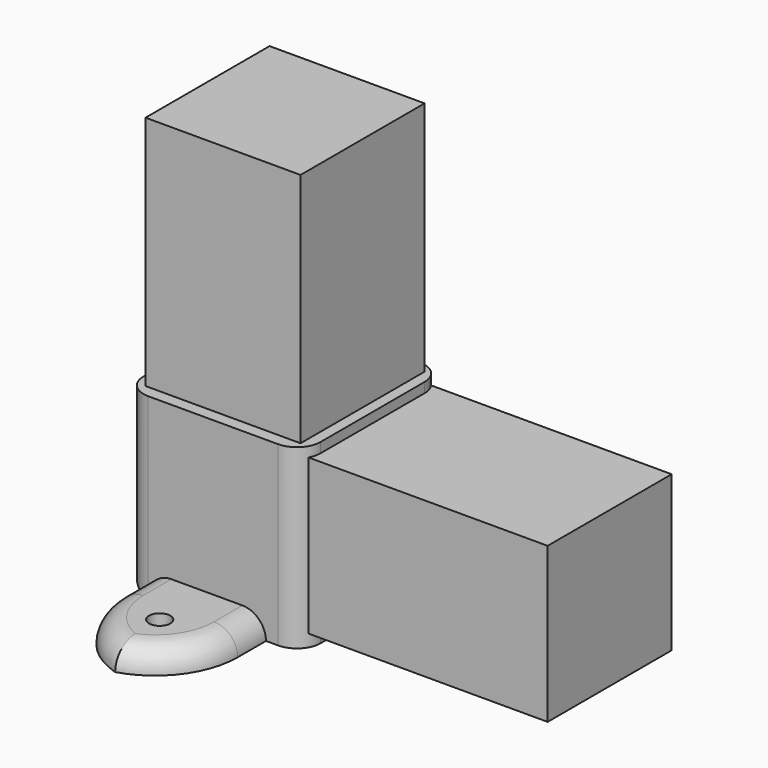
from build123d import *

# Parameters (mm, degrees)
F0_W           = 38.1
F0_H           = 38.1
F1_DEPTH       = 38.1
F2_W           = 33.3375
F2_H           = 33.3375
F3_DEPTH       = 50.8
F4_W           = 33.3375
F4_H           = 33.3375
F5_DEPTH       = 50.8
F6_W           = 25.4
F6_H           = 25.4
F7_DEPTH       = 5.08
F8_R           = 2.286
F9_DEPTH       = 83.82
F10_T1_DEPTH   = 93.9954855022
F10_2_T1_DEPTH = 93.9954855022
F11_T1_DEPTH   = 63.5
F11_T3_DEPTH   = 63.5
F11_T8_DEPTH   = 63.5
F11_T14_DEPTH  = 63.5
F11_T20_DEPTH  = 63.5
F11_T27_DEPTH  = 63.5
F11_T33_DEPTH  = 63.5
F11_T39_DEPTH  = 63.5
F11_T45_DEPTH  = 63.5
F11_T51_DEPTH  = 63.5
F11_T58_DEPTH  = 63.5
F11_T64_DEPTH  = 63.5
F11_2_T1_DEPTH = 20.3169028996
F11_2_T4_ANGLE = 114.3203710668
F11_2_T6_ANGLE = 114.3203710677
F11_3_T1_DEPTH = 20.3169028996
F11_3_T4_ANGLE = 114.3203710668
F11_3_T6_ANGLE = 114.3203710677


# Not quite as in the source:
# - a fillet or chamfer that OpenCascade refuses, or shapes differently, is made with other operations: its cross-section is extruded or revolved along the edge and cut away or added


with BuildPart() as f1:
    # F0 (on Front) → F1 (new body)
    with BuildSketch(Plane.XZ):
        with Locations((19.3985427063, -10.1599991322)):
            Rectangle(F0_W, F0_H)
    extrude(amount=F1_DEPTH)

    # F2 (on face) → F3 (join)
    with BuildSketch(Plane.YZ.offset(38.4485427063)):
        with Locations((-18.8190903282, -9.9104456074)):
            Rectangle(F2_W, F2_H)
    extrude(amount=F3_DEPTH)

    # F11: fillet of radius 5.08 on 5 edges, made by hand

    # F11_s2 → F11_t1 (cut)
    with BuildSketch(Plane.XY.offset(-41.9099991322)):
        with BuildLine():
            ThreePointArc((0.3485427063, -5.08), (1.8364402579, -1.4878975516), (5.4285427063, 0))
            Line((5.4285427063, 0), (0.3485427063, 0))
            Line((0.3485427063, 0), (0.3485427063, -5.08))
        make_face()
        with BuildLine():
            ThreePointArc((0.3485427063, -33.02), (1.8364402579, -36.6121024484), (5.4285427063, -38.1))
            Line((5.4285427063, -38.1), (0.3485427063, -38.1))
            Line((0.3485427063, -38.1), (0.3485427063, -33.02))
        make_face()
    extrude(amount=F11_T1_DEPTH, mode=Mode.SUBTRACT)

    # F11_s4 → F11_t3 (cut)
    with BuildSketch(Plane.XZ.offset(-12.7)):
        with BuildLine():
            ThreePointArc((0.3485427063, -24.1299991322), (1.8364402579, -27.7221015806), (5.4285427063, -29.2099991322))
            Line((5.4285427063, -29.2099991322), (0.3485427063, -29.2099991322))
            Line((0.3485427063, -29.2099991322), (0.3485427063, -24.1299991322))
        make_face()
    extrude(amount=F11_T3_DEPTH, mode=Mode.SUBTRACT)


with BuildPart() as f5:
    # F4 (on face) → F5 (new body)
    with BuildSketch(Plane.XY.offset(8.8900008678)):
        with Locations((19.4469346859, -18.8190890476)):
            Rectangle(F4_W, F4_H)
    extrude(amount=F5_DEPTH)


with BuildPart() as f7:
    # F6 (on face) → F7 (new body)
    with BuildSketch(Plane(origin=(0, 0, -29.2099991322), x_dir=(1, 0, 0), z_dir=(0, 0, -1))):
        with Locations((18.0697256371, -12.7)):
            Rectangle(F6_W, F6_H)
    extrude(amount=-F7_DEPTH)


with BuildPart() as f7b:
    # F6 (on face) → F7, piece 2 (new body)
    with BuildSketch(Plane(origin=(0, 0, -29.2099991322), x_dir=(1, 0, 0), z_dir=(0, 0, -1))):
        with Locations((18.0697256371, 50.8)):
            Rectangle(F6_W, F6_H)
    extrude(amount=-F7_DEPTH)


with BuildPart() as f9_tool:
    # F8 (on face) → F9 (new body)
    with BuildSketch(Plane.XY.offset(-24.1299991322)):
        with Locations((18.0697256371, -50.8)):
            Circle(F8_R)
        with Locations((18.0697256371, 12.7)):
            Circle(F8_R)
    extrude(amount=-F9_DEPTH)


with BuildPart() as f7_1:
    add(f7.part)

    # F9: cut by f9_tool
    add(f9_tool.part, mode=Mode.SUBTRACT)

    # F10: fillet of radius 17.7830971004 on 2 edges, made by hand

    # F10_s2 → F10_t1 (cut)
    with BuildSketch(Plane.XY.offset(-73.6677418833)):
        with BuildLine():
            ThreePointArc((5.3697256371, 7.6169028996), (10.5782741874, 20.1914514498), (23.1528227376, 25.4))
            Line((23.1528227376, 25.4), (5.3697256371, 25.4))
            Line((5.3697256371, 25.4), (5.3697256371, 7.6169028996))
        make_face()
        with BuildLine():
            ThreePointArc((30.7697256371, 7.6169028996), (25.5611770869, 20.1914514498), (12.9866285367, 25.4))
            Line((12.9866285367, 25.4), (30.7697256371, 25.4))
            Line((30.7697256371, 25.4), (30.7697256371, 7.6169028996))
        make_face()
    extrude(amount=F10_T1_DEPTH, mode=Mode.SUBTRACT)

    # F11#2: fillet of radius 5.08 on 2 edges, made by hand

    # F11_2_s2 → F11_2_t1 (cut)
    with BuildSketch(Plane.XZ.offset(-7.6169028996)):
        with BuildLine():
            ThreePointArc((30.7697256371, -29.2099991322), (29.2818280856, -25.6178966837), (25.6897256371, -24.1299991322))
            Line((25.6897256371, -24.1299991322), (30.7697256371, -24.1299991322))
            Line((30.7697256371, -24.1299991322), (30.7697256371, -29.2099991322))
        make_face()
        with BuildLine():
            ThreePointArc((5.3697256371, -29.2099991322), (6.8576231887, -25.6178966837), (10.4497256371, -24.1299991322))
            Line((10.4497256371, -24.1299991322), (5.3697256371, -24.1299991322))
            Line((5.3697256371, -24.1299991322), (5.3697256371, -29.2099991322))
        make_face()
    extrude(amount=F11_2_T1_DEPTH, mode=Mode.SUBTRACT)

    # F11_2_s3 → F11_2_t4 (revolve, cut)
    with BuildSketch(Plane.XZ.offset(-7.6169028995)):
        with BuildLine():
            ThreePointArc((10.4497256371, -24.1299991322), (6.8576231887, -25.6178966837), (5.3697256371, -29.2099991322))
            Line((5.3697256371, -29.2099991322), (5.3697256371, -24.1299991322))
            Line((5.3697256371, -24.1299991322), (10.4497256371, -24.1299991322))
        make_face()
    revolve(axis=Axis((23.1528227376, 7.6169028995, -24.1299991322), (0, 0, -1)), revolution_arc=F11_2_T4_ANGLE, mode=Mode.SUBTRACT)

    # F11_2_s5 → F11_2_t6 (revolve, cut)
    with BuildSketch(Plane(origin=(13.6425072573, 6.165668504, 0), x_dir=(0, 0, 1), z_dir=(-0.9112569083, -0.4118383749, 0))):
        with BuildLine():
            ThreePointArc((-24.1299991322, 14.2956604954), (-25.6178966837, 17.8877629438), (-29.2099991322, 19.3756604954))
            Line((-29.2099991322, 19.3756604954), (-24.1299991322, 19.3756604954))
            Line((-24.1299991322, 19.3756604954), (-24.1299991322, 14.2956604954))
        make_face()
    revolve(axis=Axis((12.9866285367, 7.6169028996, -24.1299991322), (0, 0, -1)), revolution_arc=F11_2_T6_ANGLE, mode=Mode.SUBTRACT)


with BuildPart() as f7b_1:
    add(f7b.part)

    # F9: cut by f9_tool
    add(f9_tool.part, mode=Mode.SUBTRACT)

    # F10#2: fillet of radius 17.7830971004 on 2 edges, made by hand

    # F10_2_s2 → F10_2_t1 (cut)
    with BuildSketch(Plane.XY.offset(-73.6677418833)):
        with BuildLine():
            ThreePointArc((23.1528227376, -63.5), (10.5782741874, -58.2914514498), (5.3697256371, -45.7169028996))
            Line((5.3697256371, -45.7169028996), (5.3697256371, -63.5))
            Line((5.3697256371, -63.5), (23.1528227376, -63.5))
        make_face()
        with BuildLine():
            ThreePointArc((12.9866285367, -63.5), (25.5611770869, -58.2914514498), (30.7697256371, -45.7169028996))
            Line((30.7697256371, -45.7169028996), (30.7697256371, -63.5))
            Line((30.7697256371, -63.5), (12.9866285367, -63.5))
        make_face()
    extrude(amount=F10_2_T1_DEPTH, mode=Mode.SUBTRACT)

    # F11#3: fillet of radius 5.08 on 2 edges, made by hand

    # F11_3_s2 → F11_3_t1 (cut)
    with BuildSketch(Plane.XZ.offset(25.4)):
        with BuildLine():
            ThreePointArc((30.7697256371, -29.2099991322), (29.2818280856, -25.6178966837), (25.6897256371, -24.1299991322))
            Line((25.6897256371, -24.1299991322), (30.7697256371, -24.1299991322))
            Line((30.7697256371, -24.1299991322), (30.7697256371, -29.2099991322))
        make_face()
        with BuildLine():
            ThreePointArc((10.4497256371, -24.1299991322), (6.8576231887, -25.6178966837), (5.3697256371, -29.2099991322))
            Line((5.3697256371, -29.2099991322), (5.3697256371, -24.1299991322))
            Line((5.3697256371, -24.1299991322), (10.4497256371, -24.1299991322))
        make_face()
    extrude(amount=F11_3_T1_DEPTH, mode=Mode.SUBTRACT)

    # F11_3_s3 → F11_3_t4 (revolve, cut)
    with BuildSketch(Plane(origin=(2.0687305768, 0.9349532839, 0), x_dir=(0, 0, 1), z_dir=(0.9112569083, 0.4118383749, 0))):
        with BuildLine():
            ThreePointArc((-24.1299991322, 63.8981615853), (-25.6178966837, 67.4902640337), (-29.2099991322, 68.9781615853))
            Line((-29.2099991322, 68.9781615853), (-24.1299991322, 68.9781615853))
            Line((-24.1299991322, 68.9781615853), (-24.1299991322, 63.8981615853))
        make_face()
    revolve(axis=Axis((23.1528227376, -45.7169028995, -24.1299991322), (0, 0, -1)), revolution_arc=F11_3_T4_ANGLE, mode=Mode.SUBTRACT)

    # F11_3_s5 → F11_3_t6 (revolve, cut)
    with BuildSketch(Plane.XZ.offset(45.7169028996)):
        with BuildLine():
            ThreePointArc((30.7697256371, -29.2099991322), (29.2818280855, -25.6178966837), (25.6897256371, -24.1299991322))
            Line((25.6897256371, -24.1299991322), (30.7697256371, -24.1299991322))
            Line((30.7697256371, -24.1299991322), (30.7697256371, -29.2099991322))
        make_face()
    revolve(axis=Axis((12.9866285367, -45.7169028996, -24.1299991322), (0, 0, -1)), revolution_arc=F11_3_T6_ANGLE, mode=Mode.SUBTRACT)


with BuildPart() as f11_tool6:
    # F11_s7 → F11_t8 (new body)
    with BuildSketch(Plane.XY.offset(-41.9099991322)):
        with BuildLine():
            ThreePointArc((38.4485427063, -5.08), (36.9606451548, -1.4878975516), (33.3685427063, 0))
            Line((33.3685427063, 0), (38.4485427063, 0))
            Line((38.4485427063, 0), (38.4485427063, -5.08))
        make_face()
    extrude(amount=F11_T8_DEPTH)

    split(bisect_by=Plane.XZ.offset(2.1503403282), keep=Keep.TOP)

    split(bisect_by=Plane.XY.offset(-26.5791956074), keep=Keep.BOTTOM)


with BuildPart() as f1_1:
    add(f1.part)

    # F11_t5: cut F11_tool6
    add(f11_tool6.part, mode=Mode.SUBTRACT)


with BuildPart() as f11_tool12:
    # F11_s13 → F11_t14 (new body)
    with BuildSketch(Plane.XY.offset(-41.9099991322)):
        with BuildLine():
            ThreePointArc((38.4485427063, -5.08), (36.9606451548, -1.4878975516), (33.3685427063, 0))
            Line((33.3685427063, 0), (38.4485427063, 0))
            Line((38.4485427063, 0), (38.4485427063, -5.08))
        make_face()
    extrude(amount=F11_T14_DEPTH)

    split(bisect_by=Plane.XZ.offset(2.1503403282), keep=Keep.BOTTOM)

    split(bisect_by=Plane.XY.offset(-26.5791956074), keep=Keep.BOTTOM)


with BuildPart() as f1_2:
    add(f1_1.part)

    # F11_t11: cut F11_tool12
    add(f11_tool12.part, mode=Mode.SUBTRACT)


with BuildPart() as f11_tool18:
    # F11_s19 → F11_t20 (new body)
    with BuildSketch(Plane.XY.offset(-41.9099991322)):
        with BuildLine():
            ThreePointArc((38.4485427063, -5.08), (36.9606451548, -1.4878975516), (33.3685427063, 0))
            Line((33.3685427063, 0), (38.4485427063, 0))
            Line((38.4485427063, 0), (38.4485427063, -5.08))
        make_face()
    extrude(amount=F11_T20_DEPTH)

    split(bisect_by=Plane.XZ.offset(2.1503403282), keep=Keep.BOTTOM)

    split(bisect_by=Plane.XY.offset(-26.5791956074), keep=Keep.TOP)

    split(bisect_by=Plane.XY.offset(6.7583043926), keep=Keep.BOTTOM)


with BuildPart() as f1_3:
    add(f1_2.part)

    # F11_t17: cut F11_tool18
    add(f11_tool18.part, mode=Mode.SUBTRACT)


with BuildPart() as f11_tool25:
    # F11_s26 → F11_t27 (new body)
    with BuildSketch(Plane.XY.offset(-41.9099991322)):
        with BuildLine():
            ThreePointArc((38.4485427063, -5.08), (36.9606451548, -1.4878975516), (33.3685427063, 0))
            Line((33.3685427063, 0), (38.4485427063, 0))
            Line((38.4485427063, 0), (38.4485427063, -5.08))
        make_face()
    extrude(amount=F11_T27_DEPTH)

    split(bisect_by=Plane.XZ.offset(2.1503403282), keep=Keep.TOP)

    split(bisect_by=Plane.XY.offset(6.7583043926), keep=Keep.TOP)


with BuildPart() as f1_4:
    add(f1_3.part)

    # F11_t24: cut F11_tool25
    add(f11_tool25.part, mode=Mode.SUBTRACT)


with BuildPart() as f11_tool31:
    # F11_s32 → F11_t33 (new body)
    with BuildSketch(Plane.XY.offset(-41.9099991322)):
        with BuildLine():
            ThreePointArc((38.4485427063, -5.08), (36.9606451548, -1.4878975516), (33.3685427063, 0))
            Line((33.3685427063, 0), (38.4485427063, 0))
            Line((38.4485427063, 0), (38.4485427063, -5.08))
        make_face()
    extrude(amount=F11_T33_DEPTH)

    split(bisect_by=Plane.XZ.offset(2.1503403282), keep=Keep.BOTTOM)

    split(bisect_by=Plane.XY.offset(6.7583043926), keep=Keep.TOP)


with BuildPart() as f1_5:
    add(f1_4.part)

    # F11_t30: cut F11_tool31
    add(f11_tool31.part, mode=Mode.SUBTRACT)


with BuildPart() as f11_tool37:
    # F11_s38 → F11_t39 (new body)
    with BuildSketch(Plane.XY.offset(-41.9099991322)):
        with BuildLine():
            ThreePointArc((38.4485427063, -33.02), (36.9606451548, -36.6121024484), (33.3685427063, -38.1))
            Line((33.3685427063, -38.1), (38.4485427063, -38.1))
            Line((38.4485427063, -38.1), (38.4485427063, -33.02))
        make_face()
    extrude(amount=F11_T39_DEPTH)

    split(bisect_by=Plane.XY.offset(-26.5791956074), keep=Keep.BOTTOM)

    split(bisect_by=Plane.XZ.offset(35.4878403282), keep=Keep.BOTTOM)


with BuildPart() as f1_6:
    add(f1_5.part)

    # F11_t36: cut F11_tool37
    add(f11_tool37.part, mode=Mode.SUBTRACT)


with BuildPart() as f11_tool43:
    # F11_s44 → F11_t45 (new body)
    with BuildSketch(Plane.XY.offset(-41.9099991322)):
        with BuildLine():
            ThreePointArc((38.4485427063, -33.02), (36.9606451548, -36.6121024484), (33.3685427063, -38.1))
            Line((33.3685427063, -38.1), (38.4485427063, -38.1))
            Line((38.4485427063, -38.1), (38.4485427063, -33.02))
        make_face()
    extrude(amount=F11_T45_DEPTH)

    split(bisect_by=Plane.XY.offset(-26.5791956074), keep=Keep.BOTTOM)

    split(bisect_by=Plane.XZ.offset(35.4878403282), keep=Keep.TOP)


with BuildPart() as f1_7:
    add(f1_6.part)

    # F11_t42: cut F11_tool43
    add(f11_tool43.part, mode=Mode.SUBTRACT)


with BuildPart() as f11_tool49:
    # F11_s50 → F11_t51 (new body)
    with BuildSketch(Plane.XY.offset(-41.9099991322)):
        with BuildLine():
            ThreePointArc((38.4485427063, -33.02), (36.9606451548, -36.6121024484), (33.3685427063, -38.1))
            Line((33.3685427063, -38.1), (38.4485427063, -38.1))
            Line((38.4485427063, -38.1), (38.4485427063, -33.02))
        make_face()
    extrude(amount=F11_T51_DEPTH)

    split(bisect_by=Plane.XY.offset(-26.5791956074), keep=Keep.TOP)

    split(bisect_by=Plane.XZ.offset(35.4878403282), keep=Keep.TOP)

    split(bisect_by=Plane.XY.offset(6.7583043926), keep=Keep.BOTTOM)


with BuildPart() as f1_8:
    add(f1_7.part)

    # F11_t48: cut F11_tool49
    add(f11_tool49.part, mode=Mode.SUBTRACT)


with BuildPart() as f11_tool56:
    # F11_s57 → F11_t58 (new body)
    with BuildSketch(Plane.XY.offset(-41.9099991322)):
        with BuildLine():
            ThreePointArc((38.4485427063, -33.02), (36.9606451548, -36.6121024484), (33.3685427063, -38.1))
            Line((33.3685427063, -38.1), (38.4485427063, -38.1))
            Line((38.4485427063, -38.1), (38.4485427063, -33.02))
        make_face()
    extrude(amount=F11_T58_DEPTH)

    split(bisect_by=Plane.XZ.offset(35.4878403282), keep=Keep.BOTTOM)

    split(bisect_by=Plane.XY.offset(6.7583043926), keep=Keep.TOP)


with BuildPart() as f1_9:
    add(f1_8.part)

    # F11_t55: cut F11_tool56
    add(f11_tool56.part, mode=Mode.SUBTRACT)


with BuildPart() as f11_tool62:
    # F11_s63 → F11_t64 (new body)
    with BuildSketch(Plane.XY.offset(-41.9099991322)):
        with BuildLine():
            ThreePointArc((38.4485427063, -33.02), (36.9606451548, -36.6121024484), (33.3685427063, -38.1))
            Line((33.3685427063, -38.1), (38.4485427063, -38.1))
            Line((38.4485427063, -38.1), (38.4485427063, -33.02))
        make_face()
    extrude(amount=F11_T64_DEPTH)

    split(bisect_by=Plane.XZ.offset(35.4878403282), keep=Keep.TOP)

    split(bisect_by=Plane.XY.offset(6.7583043926), keep=Keep.TOP)


with BuildPart() as f1_10:
    add(f1_9.part)

    # F11_t61: cut F11_tool62
    add(f11_tool62.part, mode=Mode.SUBTRACT)


solid = Compound([f5.part, f7_1.part, f7b_1.part, f1_10.part])
